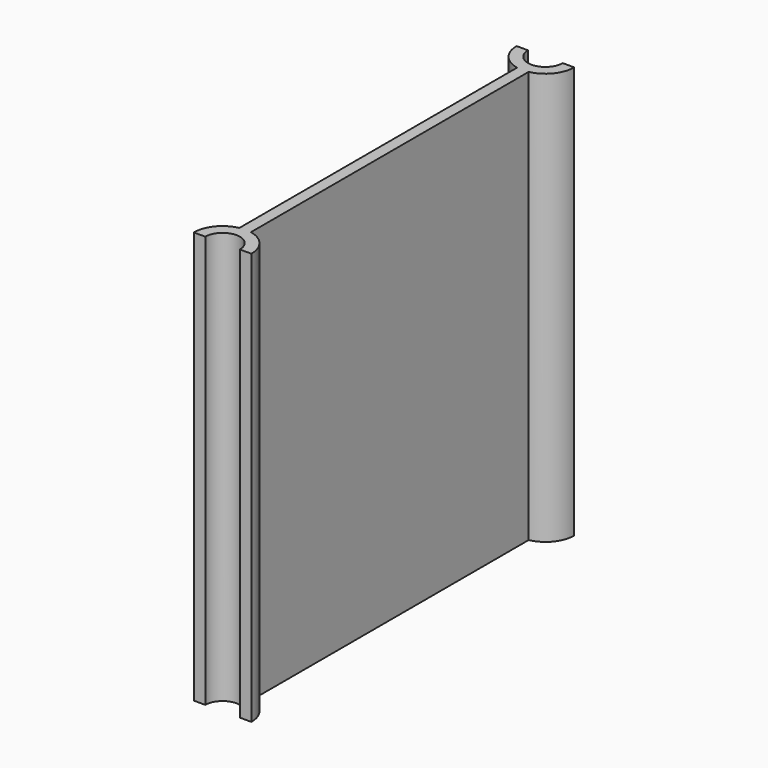
from build123d import *

# Parameters (mm, degrees)
F1_DEPTH = 35.75


# Not quite as in the source:
# - a feature names something its author has since deleted; it is built from what else it names


with BuildPart() as f1:
    # F0 (on Top) → F1 (new body)
    with BuildSketch(Plane.XY):
        with BuildLine():
            ThreePointArc((-0.5, 15.0505102572), (-0.251272405, 15.0126596175), (0, 15))
            Line((0, 15), (0, 16))
            ThreePointArc((0, 16), (-1.0606601718, 16.4393398282), (-1.5, 17.5))
            Line((-1.5, 17.5), (-2.5, 17.5))
            ThreePointArc((-2.5, 17.5), (-1.9364916731, 15.9188611699), (-0.5, 15.0505102572))
        make_face()
        with BuildLine():
            Line((0, 16), (0, 15))
            ThreePointArc((0, 15), (0.251272405, 15.0126596175), (0.5, 15.0505102572))
            ThreePointArc((0.5, 15.0505102572), (1.9364916731, 15.9188611699), (2.5, 17.5))
            Line((2.5, 17.5), (1.5, 17.5))
            ThreePointArc((1.5, 17.5), (1.0606601718, 16.4393398282), (0, 16))
        make_face()
        with BuildLine():
            ThreePointArc((0.5, 15.0505102572), (0.251272405, 15.0126596175), (0, 15))
            ThreePointArc((0, 15), (-0.251272405, 15.0126596175), (-0.5, 15.0505102572))
            Line((-0.5, 15.0505102572), (-0.5, -15.0505102572))
            ThreePointArc((-0.5, -15.0505102572), (0, -15), (0.5, -15.0505102572))
            Line((0.5, -15.0505102572), (0.5, 15.0505102572))
        make_face()
        with BuildLine():
            ThreePointArc((0.5, -15.0505102572), (0, -15), (-0.5, -15.0505102572))
            ThreePointArc((-0.5, -15.0505102572), (-1.9364916731, -15.9188611699), (-2.5, -17.5))
            Line((-2.5, -17.5), (-1.5, -17.5))
            ThreePointArc((-1.5, -17.5), (0, -16), (1.5, -17.5))
            Line((1.5, -17.5), (2.5, -17.5))
            ThreePointArc((2.5, -17.5), (1.9364916731, -15.9188611699), (0.5, -15.0505102572))
        make_face()
    extrude(amount=F1_DEPTH)


solid = f1.part
